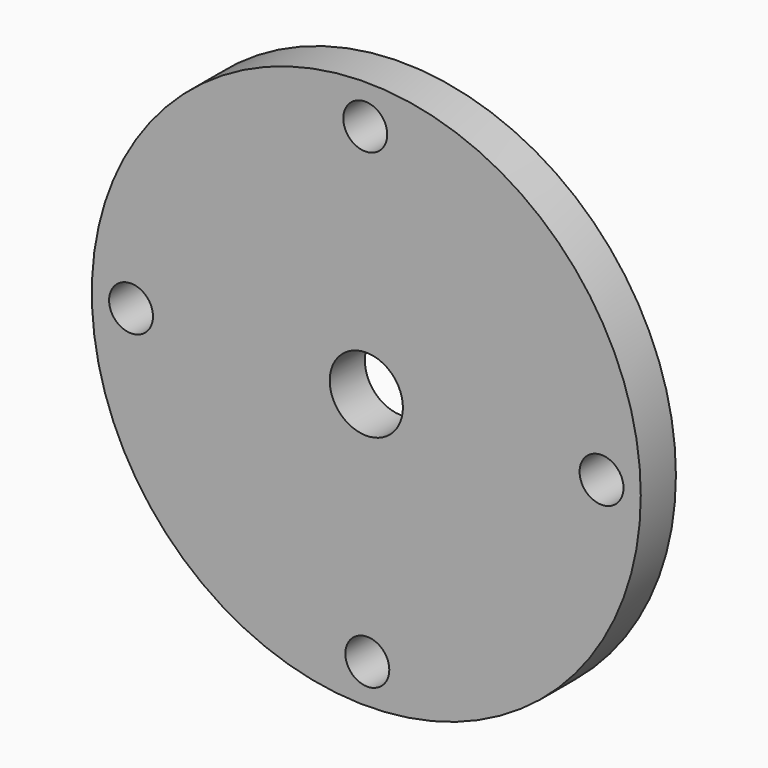
from build123d import *

# Parameters (mm, degrees)
F0_R     = 37.5
F0_R_2   = 3
F0_R_3   = 5
F1_DEPTH = 6


# Not quite as in the source:
# - a feature names something its author has since deleted; it is built from what else it names


with BuildPart() as f1:
    # F0 (on Front) → F1 (new body)
    with BuildSketch(Plane.XZ):
        with Locations((0.1399259764, 30)):
            Circle(F0_R)
        with Locations((-31.9999092322, 29.8600740236)):
            Circle(F0_R_2, mode=Mode.SUBTRACT)
        with Locations((0.2798519529, -2.1398352087)):
            Circle(F0_R_2, mode=Mode.SUBTRACT)
        with Locations((0, 62.1398352087)):
            Circle(F0_R_2, mode=Mode.SUBTRACT)
        with Locations((0.1399259764, 30)):
            Circle(F0_R_3, mode=Mode.SUBTRACT)
        with Locations((32.2797611851, 30.1399259764)):
            Circle(F0_R_2, mode=Mode.SUBTRACT)
    extrude(amount=F1_DEPTH)


solid = f1.part
